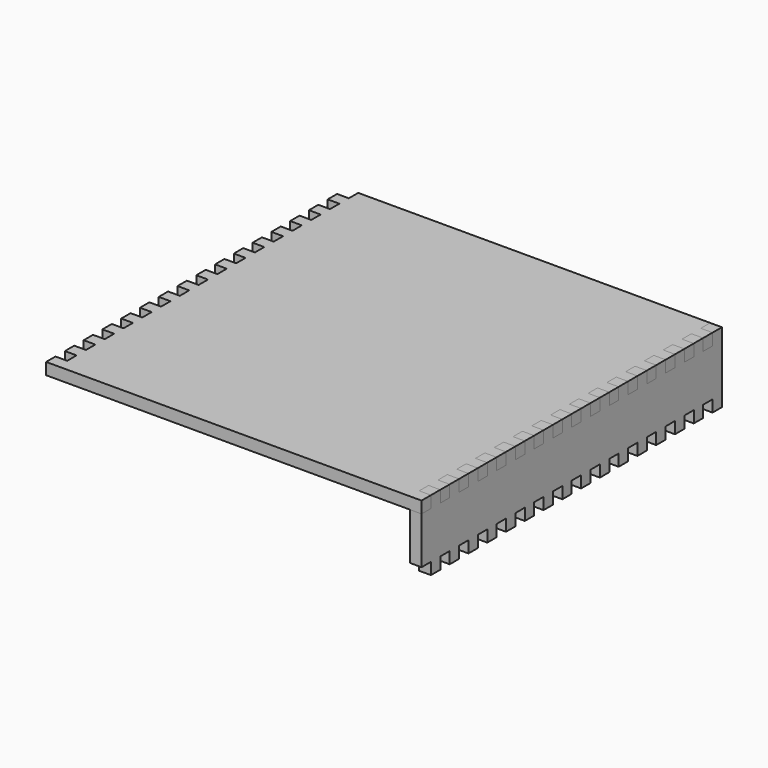
from build123d import *

# Parameters (mm, degrees)
F0_W     = 406.4
F0_H     = 406.4
F1_DEPTH = 12.7
F2_W     = 12.7
F2_H     = 12.7
F3_DEPTH = 12.7
F4_W     = 406.4
F4_H     = 76.2
F5_DEPTH = 12.7
F6_W     = 12.7
F6_H     = 12.7
F7_DEPTH = 12.7
F8_W     = 203.2
F8_H     = 76.2
F9_DEPTH = 12.7


with BuildPart() as f1:
    # F0 (on Top) → F1 (new body)
    with BuildSketch(Plane.XY):
        Rectangle(F0_W, F0_H)
    extrude(amount=F1_DEPTH)

    # F2 (on face) → F3 (cut, through all)
    with BuildSketch(Plane.XY.offset(12.7)):
        with Locations((-196.85, 196.85)):
            Rectangle(F2_W, F2_H)
        with Locations((-196.85, 171.45)):
            Rectangle(F2_W, F2_H)
        with Locations((-196.85, 146.05)):
            Rectangle(F2_W, F2_H)
        with Locations((-196.85, 120.65)):
            Rectangle(F2_W, F2_H)
        with Locations((-196.85, 95.25)):
            Rectangle(F2_W, F2_H)
        with Locations((-196.85, 69.85)):
            Rectangle(F2_W, F2_H)
        with Locations((-196.85, 44.45)):
            Rectangle(F2_W, F2_H)
        with Locations((-196.85, 19.05)):
            Rectangle(F2_W, F2_H)
        with Locations((-196.85, -6.35)):
            Rectangle(F2_W, F2_H)
        with Locations((-196.85, -31.75)):
            Rectangle(F2_W, F2_H)
        with Locations((-196.85, -57.15)):
            Rectangle(F2_W, F2_H)
        with Locations((-196.85, -82.55)):
            Rectangle(F2_W, F2_H)
        with Locations((-196.85, -107.95)):
            Rectangle(F2_W, F2_H)
        with Locations((-196.85, -133.35)):
            Rectangle(F2_W, F2_H)
        with Locations((-196.85, -158.75)):
            Rectangle(F2_W, F2_H)
        with Locations((-196.85, -184.15)):
            Rectangle(F2_W, F2_H)
        with Locations((196.85, 196.85)):
            Rectangle(F2_W, F2_H)
        with Locations((196.85, 171.45)):
            Rectangle(F2_W, F2_H)
        with Locations((196.85, 146.05)):
            Rectangle(F2_W, F2_H)
        with Locations((196.85, 120.65)):
            Rectangle(F2_W, F2_H)
        with Locations((196.85, 95.25)):
            Rectangle(F2_W, F2_H)
        with Locations((196.85, 69.85)):
            Rectangle(F2_W, F2_H)
        with Locations((196.85, 44.45)):
            Rectangle(F2_W, F2_H)
        with Locations((196.85, 19.05)):
            Rectangle(F2_W, F2_H)
        with Locations((196.85, -6.35)):
            Rectangle(F2_W, F2_H)
        with Locations((196.85, -31.75)):
            Rectangle(F2_W, F2_H)
        with Locations((196.85, -57.15)):
            Rectangle(F2_W, F2_H)
        with Locations((196.85, -82.55)):
            Rectangle(F2_W, F2_H)
        with Locations((196.85, -107.95)):
            Rectangle(F2_W, F2_H)
        with Locations((196.85, -133.35)):
            Rectangle(F2_W, F2_H)
        with Locations((196.85, -158.75)):
            Rectangle(F2_W, F2_H)
        with Locations((196.85, -184.15)):
            Rectangle(F2_W, F2_H)
    extrude(amount=-F3_DEPTH, mode=Mode.SUBTRACT)


with BuildPart() as f5:
    # F4 (on face) → F5 (new body)
    with BuildSketch(Plane.YZ.offset(203.2)):
        with Locations((0, -25.4)):
            Rectangle(F4_W, F4_H)
    extrude(amount=-F5_DEPTH)

    # F6 (on face) → F7 (cut, through all)
    with BuildSketch(Plane.YZ.offset(203.2)):
        with Locations((-196.85, 6.35)):
            Rectangle(F6_W, F6_H)
        with Locations((-196.85, -57.15)):
            Rectangle(F6_W, F6_H)
        with Locations((-171.45, 6.35)):
            Rectangle(F6_W, F6_H)
        with Locations((-171.45, -57.15)):
            Rectangle(F6_W, F6_H)
        with Locations((-146.05, 6.35)):
            Rectangle(F6_W, F6_H)
        with Locations((-146.05, -57.15)):
            Rectangle(F6_W, F6_H)
        with Locations((-120.65, 6.35)):
            Rectangle(F6_W, F6_H)
        with Locations((-120.65, -57.15)):
            Rectangle(F6_W, F6_H)
        with Locations((-95.25, 6.35)):
            Rectangle(F6_W, F6_H)
        with Locations((-95.25, -57.15)):
            Rectangle(F6_W, F6_H)
        with Locations((-69.85, 6.35)):
            Rectangle(F6_W, F6_H)
        with Locations((-69.85, -57.15)):
            Rectangle(F6_W, F6_H)
        with Locations((-44.45, 6.35)):
            Rectangle(F6_W, F6_H)
        with Locations((-44.45, -57.15)):
            Rectangle(F6_W, F6_H)
        with Locations((-19.05, 6.35)):
            Rectangle(F6_W, F6_H)
        with Locations((-19.05, -57.15)):
            Rectangle(F6_W, F6_H)
        with Locations((6.35, 6.35)):
            Rectangle(F6_W, F6_H)
        with Locations((6.35, -57.15)):
            Rectangle(F6_W, F6_H)
        with Locations((31.75, 6.35)):
            Rectangle(F6_W, F6_H)
        with Locations((31.75, -57.15)):
            Rectangle(F6_W, F6_H)
        with Locations((57.15, 6.35)):
            Rectangle(F6_W, F6_H)
        with Locations((57.15, -57.15)):
            Rectangle(F6_W, F6_H)
        with Locations((82.55, 6.35)):
            Rectangle(F6_W, F6_H)
        with Locations((82.55, -57.15)):
            Rectangle(F6_W, F6_H)
        with Locations((107.95, 6.35)):
            Rectangle(F6_W, F6_H)
        with Locations((107.95, -57.15)):
            Rectangle(F6_W, F6_H)
        with Locations((133.35, 6.35)):
            Rectangle(F6_W, F6_H)
        with Locations((133.35, -57.15)):
            Rectangle(F6_W, F6_H)
        with Locations((158.75, 6.35)):
            Rectangle(F6_W, F6_H)
        with Locations((158.75, -57.15)):
            Rectangle(F6_W, F6_H)
        with Locations((184.15, 6.35)):
            Rectangle(F6_W, F6_H)
        with Locations((184.15, -57.15)):
            Rectangle(F6_W, F6_H)
    extrude(amount=-F7_DEPTH, mode=Mode.SUBTRACT)


with BuildPart() as f9:
    # F8 (on face) → F9 (new body)
    with BuildSketch(Plane(origin=(0, 0, -63.5), x_dir=(1, 0, 0), z_dir=(0, 0, -1))):
        with Locations((0, -88.9)):
            Rectangle(F8_W, F8_H)
    extrude(amount=F9_DEPTH)


solid = Compound([f1.part, f5.part, f9.part])
